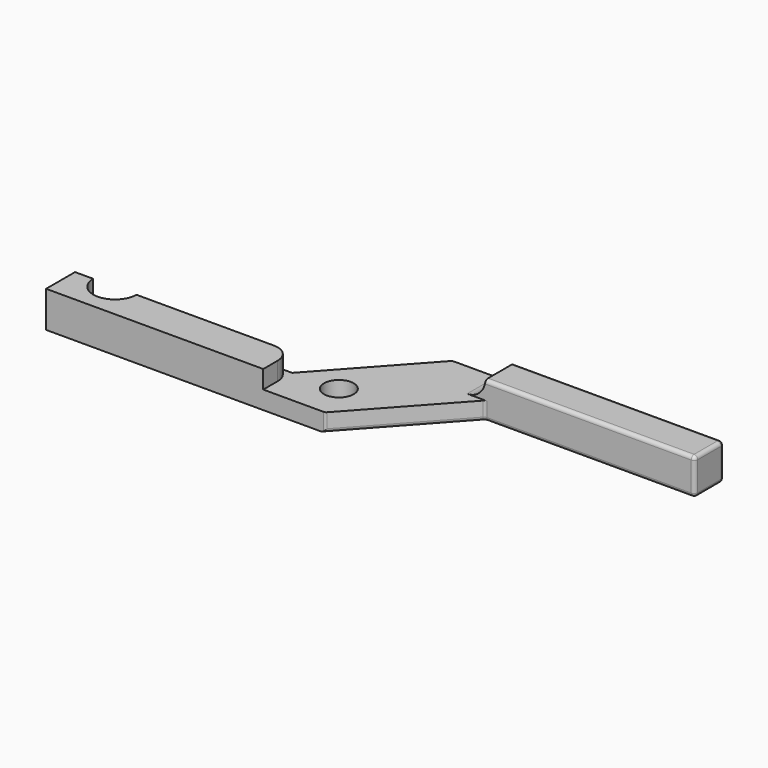
from build123d import *

# Parameters (mm, degrees)
F1_DEPTH = 10
F2_R     = 4.1
F3_DEPTH = 5
F4_DEPTH = 10
F5_R     = 1
F6_R     = 4.99999
F7_R     = 5


# Not quite as in the source:
# - a fillet or chamfer is up to 0.001 mm smaller than in the source, because OpenCascade refuses the exact size


with BuildPart() as f1:
    # F0 (on Top) → F1 (new body)
    with BuildSketch(Plane.XY):
        with BuildLine():
            Line((23.4835705605, 25.9523007406), (0, 0))
            Line((0, 0), (-43.0009548823, 0))
            ThreePointArc((-43.0009548823, 0), (-49.0004774411, -5.9243094089), (-55, 0))
            Line((-55, 0), (-60, 0))
            Line((-60, 0), (-60, -10))
            Line((-60, -10), (17.0862320811, -10))
            Line((17.0862320811, -10), (40.5698026416, 15.9523007406))
            Line((40.5698026416, 15.9523007406), (98.4835705605, 15.9523007406))
            Line((98.4835705605, 15.9523007406), (98.4835705605, 25.9523007406))
            Line((98.4835705605, 25.9523007406), (23.4835705605, 25.9523007406))
        make_face()
    extrude(amount=F1_DEPTH)

    # F2 (on face) → F3 (cut)
    with BuildSketch(Plane.XY.offset(10)):
        Polygon((0, -10), (17.0862320811, -10), (40.5698026416, 15.9523007406), (40.5698026416, 25.9523007406), (23.4835705605, 25.9523007406), (0, 0), align=None)
        with Locations((12.5, 0.5)):
            Circle(F2_R, mode=Mode.SUBTRACT)
    extrude(amount=-F3_DEPTH, mode=Mode.SUBTRACT)

    # F4 (cut, through all): a face of the model
    f4_faces = [f1.faces().sort_by_distance(p)[0] for p in [
        (12.5, 0.5, 10),
    ]]
    extrude(f4_faces, amount=-F4_DEPTH, mode=Mode.SUBTRACT)

    # F5
    f5_edges = [f1.edges().sort_by_distance(p)[0] for p in [
        (60.983571, 25.952301, 0),
        (69.526687, 25.952301, 10),
        (98.483571, 25.952301, 5),
        (98.483571, 20.952301, 0),
        (98.483571, 20.952301, 10),
        (98.483571, 15.952301, 5),
        (69.526687, 15.952301, 0),
        (69.526687, 15.952301, 10),
        (23.483571, 25.952301, 2.5),
        (17.086232, -10, 2.5),
        (40.569803, 15.952301, 2.5),
        (28.828017, 2.97615, 0),
    ]]
    fillet(f5_edges, radius=F5_R)

    # F6 (radius 5 in the source; OpenCascade refuses exactly that, so slightly less here)
    f6_edges = [f1.edges().sort_by_distance(p)[0] for p in [
        (40.569803, 20.952301, 5),
    ]]
    fillet(f6_edges, radius=F6_R)

    # F7
    f7_edges = [f1.edges().sort_by_distance(p)[0] for p in [
        (0, 0, 7.5),
    ]]
    fillet(f7_edges, radius=F7_R)


solid = f1.part
